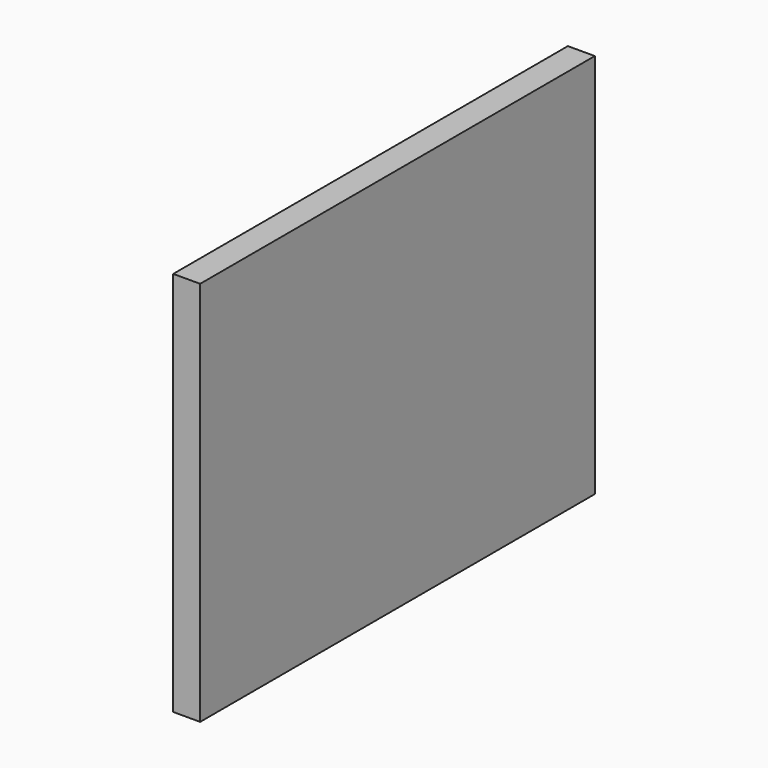
from build123d import *

# Parameters (mm, degrees)
F1_DEPTH = 3


# Not quite as in the source:
# - ends of sketch curves that miss each other by under 0.0002 mm in the source are joined


with BuildPart() as f1:
    # F0 (on Right) → F1 (new body)
    with BuildSketch(Plane.YZ):
        Polygon((-27.499976, 19.999999), (-27.499976, -19.999998), (27.499976, -19.999998), (27.500024, 19.999999), (27.499976, 23.000002), (-27.499976, 23.000002), align=None)
    extrude(amount=F1_DEPTH)


solid = f1.part
